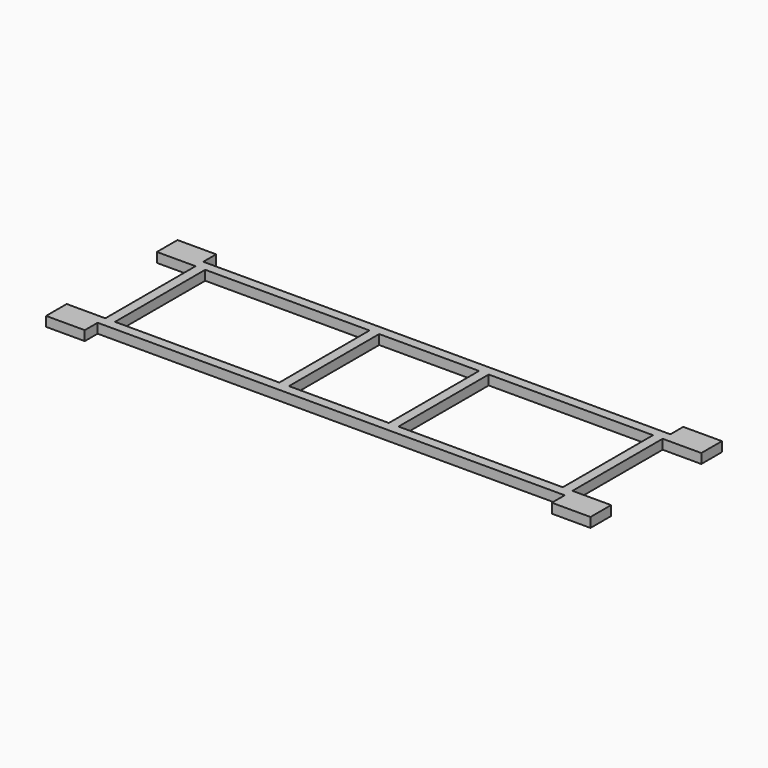
from build123d import *

# Parameters (mm, degrees)
F0_W     = 169
F0_H     = 51
F1_DEPTH = 3
F2_W     = 51
F2_H     = 35
F2_W_2   = 12
F2_W_3   = 72.5
F2_H_2   = 5
F2_W_4   = 15.5
F3_DEPTH = 3


# Not quite as in the source:
# - a pattern or mirror of a feature is missing from the dataset's text; its kind, count and spacing are read off the source's solid


with BuildPart() as f1:
    # F0 (on Top) → F1 (new body)
    with BuildSketch(Plane.XY):
        Rectangle(F0_W, F0_H)
    extrude(amount=F1_DEPTH)

    # F2 (on face) → F3 (cut, through all)
    with BuildSketch(Plane.XY.offset(3)):
        with Locations((-44, 0)):
            Rectangle(F2_W, F2_H)
        with Locations((-78.5, 0)):
            Rectangle(F2_W_2, F2_H)
        with Locations((-36.25, 23)):
            Rectangle(F2_W_3, F2_H_2)
        with Locations((-36.25, -23)):
            Rectangle(F2_W_3, F2_H_2)
        with Locations((-7.75, 0)):
            Rectangle(F2_W_4, F2_H)
    f3 = extrude(amount=-F3_DEPTH, mode=Mode.SUBTRACT)

    # F3_copies: F3 across plane
    add(f3.mirror(Plane(origin=(0, 0, 0), x_dir=(0, 0, 1), z_dir=(1, 0, 0))), mode=Mode.SUBTRACT)


solid = f1.part
